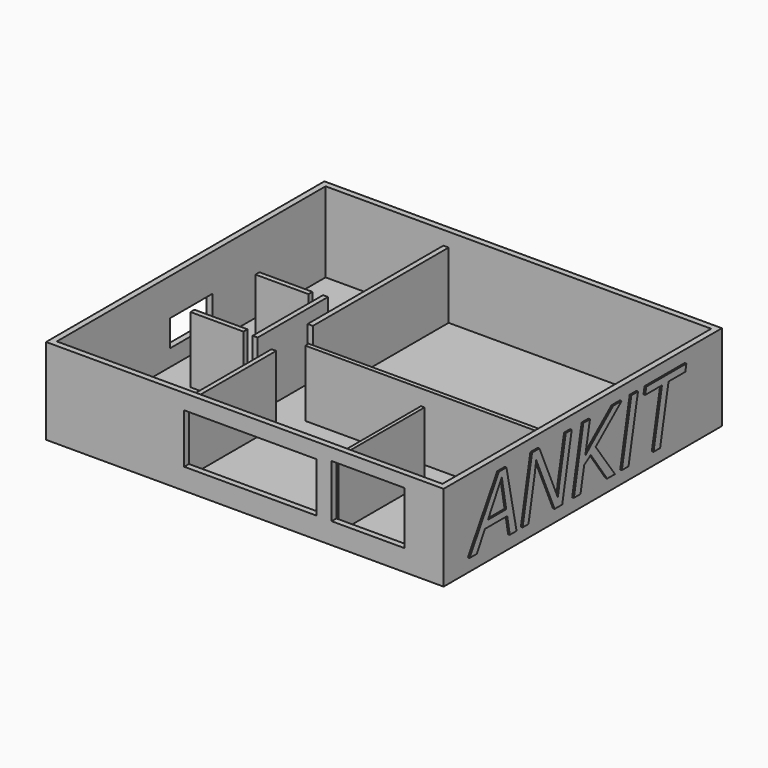
from build123d import *

# Parameters (mm, degrees)
F0_W          = 120
F0_H          = 105
F1_DEPTH      = 26
F2_T          = -1.8
F3_W          = 22
F3_H          = 16
F3_W_2        = 40
F3_H_2        = 15
F4_DEPTH      = 1.8
F5_W          = 70.7417093217
F5_H          = 1.2750467286
F5_W_2        = 1.0632928461
F5_H_2        = 32.3836449534
F5_W_3        = 1.3958998024
F5_H_3        = 33.5804019123
F6_DEPTH      = 20
F7_W          = 16
F7_H          = 1.5
F7_W_2        = 1.5
F7_H_2        = 26.5304031223
F7_W_3        = 1.5820730478
F7_H_3        = 51.2154798855
F8_DEPTH      = 20
F9_W          = 16
F9_H          = 8
F10_DEPTH     = 1.8
F11_TEXT_SIZE = 26.8008534072
F13_DEPTH     = 0.5
F12_TEXT_SIZE = 21.9472193231
F14_DEPTH     = 0.5


# Not quite as in the source:
# - Text() gives the source's letters only with a copy of the font that has no kerning and outlines rounded to 1/6400 em; it was checked with that copy


with BuildPart() as f1:
    # F0 (on Top) → F1 (new body)
    with BuildSketch(Plane.XY):
        Rectangle(F0_W, F0_H)
    extrude(amount=F1_DEPTH)

    # F2
    f2_openings = [f1.faces().sort_by_distance(p)[0] for p in [
        (0, 0, 26),
    ]]
    offset(amount=F2_T, openings=f2_openings)

    # F3 (on face) → F4 (cut, through all)
    with BuildSketch(Plane.XZ.offset(52.5)):
        with Locations((37.2, 14.4)):
            Rectangle(F3_W, F3_H)
        with Locations((1.7, 13.9)):
            Rectangle(F3_W_2, F3_H_2)
    extrude(amount=-F4_DEPTH, mode=Mode.SUBTRACT)

    # F5 (on face) → F6 (join)
    with BuildSketch(Plane.XY.offset(1.8)):
        with Locations((19.2058440298, -8.8583952747)):
            Rectangle(F5_W, F5_H)
        with Locations((24.9491175637, -32.7740302309)):
            Rectangle(F5_W_2, F5_H_2)
        with Locations((-20.5446593463, -32.6739093289)):
            Rectangle(F5_W_3, F5_H_3)
    extrude(amount=F6_DEPTH)

    # F7 (on face) → F8 (join)
    with BuildSketch(Plane.XY.offset(1.8)):
        with Locations((-40, 12.25)):
            Rectangle(F7_W, F7_H)
        with Locations((-28.25, -0.0347984388)):
            Rectangle(F7_W_2, F7_H_2)
        with Locations((-40, -12.25)):
            Rectangle(F7_W, F7_H)
        with Locations((-21.8489402905, 25.0922600572)):
            Rectangle(F7_W_3, F7_H_3)
    extrude(amount=F8_DEPTH)

    # F9 (on face) → F10 (cut, through all)
    with BuildSketch(Plane(origin=(-60, 0, 0), x_dir=(0, -1, 0), z_dir=(-1, 0, 0))):
        with Locations((0, 10.8)):
            Rectangle(F9_W, F9_H)
    extrude(amount=-F10_DEPTH, mode=Mode.SUBTRACT)

    # F11 (on face) → F13 (join)
    with BuildSketch(Plane.YZ.offset(60)):
        with Locations((-42.0457161963, 4.0369015187)):
            Text('ANKIT', F11_TEXT_SIZE, font='Arimo', font_style=FontStyle.ITALIC, text_align=(TextAlign.LEFT, TextAlign.BOTTOM))
    extrude(amount=F13_DEPTH)

    # F12 (on face) → F14 (join)
    with BuildSketch(Plane(origin=(0, 52.5, 0), x_dir=(-1, 0, 0), z_dir=(0, 1, 0))):
        with Locations((-57.8435012602, 5.3557090191)):
            Text('BADATALA', F12_TEXT_SIZE, font='Arimo', font_style=FontStyle.ITALIC, text_align=(TextAlign.LEFT, TextAlign.BOTTOM))
    extrude(amount=F14_DEPTH)


solid = f1.part
